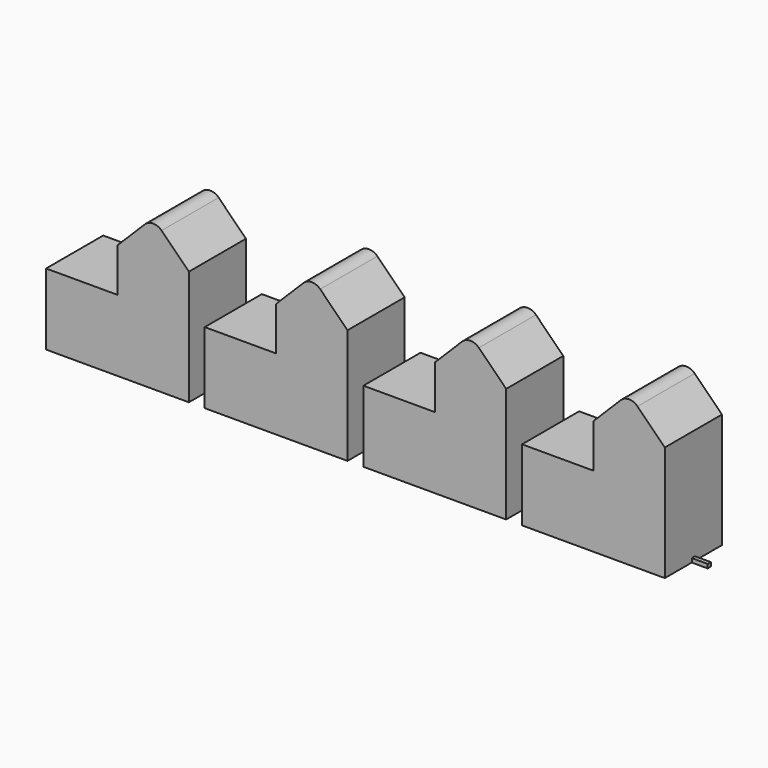
from build123d import *

# Parameters (mm, degrees)
F1_DEPTH = 9
F2_W     = 2
F2_H     = 4.25
F3_DEPTH = 18.3796796564


# Not quite as in the source:
# - a feature names something its author has since deleted; it is built from what else it names


with BuildPart() as f1:
    # F0 (on Front) → F1 (new body)
    with BuildSketch(Plane.XZ):
        with BuildLine():
            Line((-9, -4.5), (9, -4.5))
            Line((9, -4.5), (11, -4.5))
            Line((11, -4.5), (11, -4))
            Line((11, -4), (9, -4))
            Line((9, -4), (9, 4.5))
            Line((9, 4.5), (9, 10))
            Line((9, 10), (5.5606601718, 13.4393398282))
            ThreePointArc((5.5606601718, 13.4393398282), (4.5, 13.8786796564), (3.4393398282, 13.4393398282))
            Line((3.4393398282, 13.4393398282), (0, 10))
            Line((0, 10), (0, 4.5))
            Line((0, 4.5), (-9, 4.5))
            Line((-9, 4.5), (-9, -4.5))
        make_face()
        with BuildLine():
            Line((11, -4), (11, -4.5))
            Line((11, -4.5), (29, -4.5))
            Line((29, -4.5), (31, -4.5))
            Line((31, -4.5), (31, -4))
            Line((31, -4), (29, -4))
            Line((29, -4), (29, 4.5))
            Line((29, 4.5), (29, 10))
            Line((29, 10), (25.5606601718, 13.4393398282))
            ThreePointArc((25.5606601718, 13.4393398282), (24.5, 13.8786796564), (23.4393398282, 13.4393398282))
            Line((23.4393398282, 13.4393398282), (20, 10))
            Line((20, 10), (20, 4.5))
            Line((20, 4.5), (11, 4.5))
            Line((11, 4.5), (11, -4))
        make_face()
        with BuildLine():
            Line((31, -4), (31, -4.5))
            Line((31, -4.5), (49, -4.5))
            Line((49, -4.5), (51, -4.5))
            Line((51, -4.5), (51, -4))
            Line((51, -4), (49, -4))
            Line((49, -4), (49, 4.5))
            Line((49, 4.5), (49, 10))
            Line((49, 10), (45.5606601718, 13.4393398282))
            ThreePointArc((45.5606601718, 13.4393398282), (44.5, 13.8786796564), (43.4393398282, 13.4393398282))
            Line((43.4393398282, 13.4393398282), (40, 10))
            Line((40, 10), (40, 4.5))
            Line((40, 4.5), (31, 4.5))
            Line((31, 4.5), (31, -4))
        make_face()
        with BuildLine():
            Line((51, -4), (51, -4.5))
            Line((51, -4.5), (69, -4.5))
            Line((69, -4.5), (71, -4.5))
            Line((71, -4.5), (71, -4))
            Line((71, -4), (69, -4))
            Line((69, -4), (69, 4.5))
            Line((69, 4.5), (69, 10))
            Line((69, 10), (65.5606601718, 13.4393398282))
            ThreePointArc((65.5606601718, 13.4393398282), (64.5, 13.8786796564), (63.4393398282, 13.4393398282))
            Line((63.4393398282, 13.4393398282), (60, 10))
            Line((60, 10), (60, 4.5))
            Line((60, 4.5), (51, 4.5))
            Line((51, 4.5), (51, -4))
        make_face()
    extrude(amount=-F1_DEPTH)

    # F2 (on face) → F3 (cut, through all)
    with BuildSketch(Plane(origin=(0, 0, -4.5), x_dir=(1, 0, 0), z_dir=(0, 0, -1))):
        with Locations((10, -2.125)):
            Rectangle(F2_W, F2_H)
        with Locations((10, -6.875)):
            Rectangle(F2_W, F2_H)
        with Locations((30, -2.125)):
            Rectangle(F2_W, F2_H)
        with Locations((30, -6.875)):
            Rectangle(F2_W, F2_H)
        with Locations((50, -2.125)):
            Rectangle(F2_W, F2_H)
        with Locations((50, -6.875)):
            Rectangle(F2_W, F2_H)
        with Locations((70, -2.125)):
            Rectangle(F2_W, F2_H)
        with Locations((70, -6.875)):
            Rectangle(F2_W, F2_H)
    extrude(amount=-F3_DEPTH, mode=Mode.SUBTRACT)


solid = f1.part
